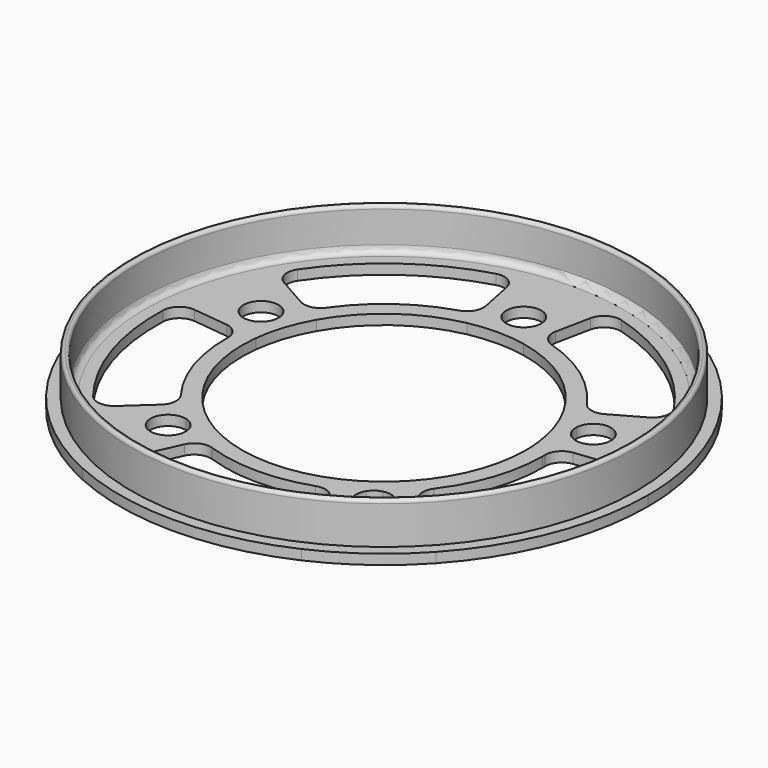
from build123d import *

# Parameters (mm, degrees)
F1_DEPTH = 3
F2_R     = 5
F3_R     = 75.6
F3_R_2   = 73.6
F4_DEPTH = 12.4
F5_R     = 0.99999
F6_R     = 2


# Not quite as in the source:
# - a fillet or chamfer is up to 0.001 mm smaller than in the source, because OpenCascade refuses the exact size


with BuildPart() as f1:
    # F0 (on Top) → F1 (new body)
    with BuildSketch(Plane.XY):
        with BuildLine():
            ThreePointArc((-13.5579196876, 66.6346967709), (0, 68), (13.5579196876, 66.6346967709))
            Line((13.5579196876, 66.6346967709), (15.7511125782, 77.4138388956))
            ThreePointArc((15.7511125782, 77.4138388956), (0, 79), (-15.7511125782, 77.4138388956))
            Line((-15.7511125782, 77.4138388956), (-13.5579196876, 66.6346967709))
        make_face()
        with BuildLine():
            ThreePointArc((13.5579196876, 66.6346967709), (39.9693971559, 55.0131556175), (59.1837349834, 33.4856015835))
            Line((59.1837349834, 33.4856015835), (68.7575744661, 38.902390075))
            ThreePointArc((68.7575744661, 38.902390075), (46.4350349311, 63.9123425556), (15.7511125782, 77.4138388956))
            Line((15.7511125782, 77.4138388956), (13.5579196876, 66.6346967709))
        make_face()
        with BuildLine():
            ThreePointArc((8.4736998047, 41.6466854818), (24.9808732224, 34.3832222609), (36.9898343647, 20.9285009897))
            Line((36.9898343647, 20.9285009897), (41.341579584, 23.3906775767))
            ThreePointArc((41.341579584, 23.3906775767), (27.9197994839, 38.4283072328), (9.4706056641, 46.5462955385))
            Line((9.4706056641, 46.5462955385), (8.4736998047, 41.6466854818))
        make_face()
        with BuildLine():
            ThreePointArc((-8.4736998047, 41.6466854818), (0, 42.5), (8.4736998047, 41.6466854818))
            Line((8.4736998047, 41.6466854818), (9.4706056641, 46.5462955385))
            ThreePointArc((9.4706056641, 46.5462955385), (5.7500684223, 47.1506809404), (1.9933228139, 47.4581569823))
            ThreePointArc((1.9933228139, 47.4581569823), (0, 47.0650247137), (-1.9933228139, 47.4581569823))
            ThreePointArc((-1.9933228139, 47.4581569823), (-5.7500684223, 47.1506809404), (-9.4706056641, 46.5462955385))
            Line((-9.4706056641, 46.5462955385), (-8.4736998047, 41.6466854818))
        make_face()
        with BuildLine():
            ThreePointArc((1.9933228139, 47.4581569823), (5.7500684223, 47.1506809404), (9.4706056641, 46.5462955385))
            Line((9.4706056641, 46.5462955385), (13.5579196876, 66.6346967709))
            ThreePointArc((13.5579196876, 66.6346967709), (0, 68), (-13.5579196876, 66.6346967709))
            Line((-13.5579196876, 66.6346967709), (-9.4706056641, 46.5462955385))
            ThreePointArc((-9.4706056641, 46.5462955385), (-5.7500684223, 47.1506809404), (-1.9933228139, 47.4581569823))
            ThreePointArc((-1.9933228139, 47.4581569823), (-2.9238292723, 56.6754974388), (5.25, 52.3150247137))
            ThreePointArc((5.25, 52.3150247137), (4.3604727251, 49.3911954414), (1.9933228139, 47.4581569823))
        make_face()
        with BuildLine():
            ThreePointArc((45.7513600742, 12.769614378), (46.6198312174, 9.1017216648), (47.1947357785, 5.3765151165))
            Line((47.1947357785, 5.3765151165), (67.5629901671, 7.6969058509))
            ThreePointArc((67.5629901671, 7.6969058509), (64.6718431081, 21.0131556175), (59.1837349834, 33.4856015835))
            Line((59.1837349834, 33.4856015835), (41.341579584, 23.3906775767))
            ThreePointArc((41.341579584, 23.3906775767), (43.0660934948, 20.039001749), (44.5194188246, 16.5611396805))
            ThreePointArc((44.5194188246, 16.5611396805), (49.952139145, 21.4125119623), (55.0045451541, 16.1662316977))
            ThreePointArc((55.0045451541, 16.1662316977), (51.5636579657, 11.2377825669), (45.7513600742, 12.769614378))
        make_face()
        with BuildLine():
            ThreePointArc((36.9898343647, 20.9285009897), (40.4199019425, 13.1332222609), (42.2268688544, 4.8105661568))
            Line((42.2268688544, 4.8105661568), (47.1947357785, 5.3765151165))
            ThreePointArc((47.1947357785, 5.3765151165), (46.6198312174, 9.1017216648), (45.7513600742, 12.769614378))
            ThreePointArc((45.7513600742, 12.769614378), (44.7614984435, 14.5438924772), (44.5194188246, 16.5611396805))
            ThreePointArc((44.5194188246, 16.5611396805), (43.0660934948, 20.039001749), (41.341579584, 23.3906775767))
            Line((41.341579584, 23.3906775767), (36.9898343647, 20.9285009897))
        make_face()
        with BuildLine():
            ThreePointArc((59.1837349834, 33.4856015835), (64.6718431081, 21.0131556175), (67.5629901671, 7.6969058509))
            Line((67.5629901671, 7.6969058509), (78.4922974, 8.9419935621))
            ThreePointArc((78.4922974, 8.9419935621), (75.1334647873, 24.4123425556), (68.7575744661, 38.902390075))
            Line((68.7575744661, 38.902390075), (59.1837349834, 33.4856015835))
        make_face()
        with BuildLine():
            Line((78.4922974, 8.9419935621), (67.5629901671, 7.6969058509))
            ThreePointArc((67.5629901671, 7.6969058509), (67.890659635, 3.8546509982), (68, 0))
            ThreePointArc((68, 0), (63.3767015757, -24.6453585365), (50.1354794885, -45.9394568585))
            Line((50.1354794885, -45.9394568585), (58.2456305823, -53.3708395856))
            ThreePointArc((58.2456305823, -53.3708395856), (73.6288150658, -28.6321077115), (79, 0))
            ThreePointArc((79, 0), (78.8729722231, 4.4781974832), (78.4922974, 8.9419935621))
        make_face()
        with BuildLine():
            ThreePointArc((42.2268688544, 4.8105661568), (42.4316622719, 2.4091568739), (42.5, 0))
            ThreePointArc((42.5, 0), (39.6104384848, -15.4033490853), (31.3346746803, -28.7121605366))
            Line((31.3346746803, -28.7121605366), (35.0211069957, -32.0900617762))
            ThreePointArc((35.0211069957, -32.0900617762), (44.2704900712, -17.2155078012), (47.5, 0))
            ThreePointArc((47.5, 0), (47.4236225392, 2.6925870943), (47.1947357785, 5.3765151165))
            Line((47.1947357785, 5.3765151165), (42.2268688544, 4.8105661568))
        make_face()
        with BuildLine():
            Line((35.0211069957, -32.0900617762), (31.3346746803, -28.7121605366))
            ThreePointArc((31.3346746803, -28.7121605366), (24.9808732224, -34.3832222609), (17.6239403858, -38.6735920917))
            Line((17.6239403858, -38.6735920917), (19.6973451371, -43.2234264555))
            ThreePointArc((19.6973451371, -43.2234264555), (23.0625718199, -41.5255075954), (26.2825727435, -39.5661012735))
            ThreePointArc((26.2825727435, -39.5661012735), (27.6641274255, -38.076404834), (29.5078368069, -37.2228097673))
            ThreePointArc((29.5078368069, -37.2228097673), (32.3663779647, -34.7658967588), (35.0211069957, -32.0900617762))
        make_face()
        with BuildLine():
            Line((19.6973451371, -43.2234264555), (17.6239403858, -38.6735920917))
            ThreePointArc((17.6239403858, -38.6735920917), (0, -42.5), (-17.6239403858, -38.6735920917))
            Line((-17.6239403858, -38.6735920917), (-19.6973451371, -43.2234264555))
            ThreePointArc((-19.6973451371, -43.2234264555), (0, -47.5), (19.6973451371, -43.2234264555))
        make_face()
        with BuildLine():
            ThreePointArc((-17.6239403858, -38.6735920917), (-24.9808732224, -34.3832222609), (-31.3346746803, -28.7121605366))
            Line((-31.3346746803, -28.7121605366), (-35.0211069957, -32.0900617762))
            ThreePointArc((-35.0211069957, -32.0900617762), (-32.3663779647, -34.7658967588), (-29.5078368069, -37.2228097673))
            ThreePointArc((-29.5078368069, -37.2228097673), (-27.6641274255, -38.076404834), (-26.2825727435, -39.5661012735))
            ThreePointArc((-26.2825727435, -39.5661012735), (-23.0625718199, -41.5255075954), (-19.6973451371, -43.2234264555))
            Line((-19.6973451371, -43.2234264555), (-17.6239403858, -38.6735920917))
        make_face()
        with BuildLine():
            Line((-35.0211069957, -32.0900617762), (-31.3346746803, -28.7121605366))
            ThreePointArc((-31.3346746803, -28.7121605366), (-40.4199019425, -13.1332222609), (-42.2268688544, 4.8105661568))
            Line((-42.2268688544, 4.8105661568), (-47.1947357785, 5.3765151165))
            ThreePointArc((-47.1947357785, 5.3765151165), (-45.175184524, -14.6783072328), (-35.0211069957, -32.0900617762))
        make_face()
        with BuildLine():
            ThreePointArc((-42.2268688544, 4.8105661568), (-40.4199019425, 13.1332222609), (-36.9898343647, 20.9285009897))
            Line((-36.9898343647, 20.9285009897), (-41.341579584, 23.3906775767))
            ThreePointArc((-41.341579584, 23.3906775767), (-43.0660934948, 20.039001749), (-44.5194188246, 16.5611396805))
            ThreePointArc((-44.5194188246, 16.5611396805), (-44.5082648895, 16.3638256886), (-44.5045451541, 16.1662316977))
            ThreePointArc((-44.5045451541, 16.1662316977), (-44.8260960233, 14.357118886), (-45.7513600742, 12.769614378))
            ThreePointArc((-45.7513600742, 12.769614378), (-46.6198312174, 9.1017216648), (-47.1947357785, 5.3765151165))
            Line((-47.1947357785, 5.3765151165), (-42.2268688544, 4.8105661568))
        make_face()
        with BuildLine():
            Line((-41.341579584, 23.3906775767), (-36.9898343647, 20.9285009897))
            ThreePointArc((-36.9898343647, 20.9285009897), (-24.9808732224, 34.3832222609), (-8.4736998047, 41.6466854818))
            Line((-8.4736998047, 41.6466854818), (-9.4706056641, 46.5462955385))
            ThreePointArc((-9.4706056641, 46.5462955385), (-27.9197994839, 38.4283072328), (-41.341579584, 23.3906775767))
        make_face()
        with BuildLine():
            ThreePointArc((-44.5194188246, 16.5611396805), (-43.0660934948, 20.039001749), (-41.341579584, 23.3906775767))
            Line((-41.341579584, 23.3906775767), (-59.1837349834, 33.4856015835))
            ThreePointArc((-59.1837349834, 33.4856015835), (-64.6718431081, 21.0131556175), (-67.5629901671, 7.6969058509))
            Line((-67.5629901671, 7.6969058509), (-47.1947357785, 5.3765151165))
            ThreePointArc((-47.1947357785, 5.3765151165), (-46.6198312174, 9.1017216648), (-45.7513600742, 12.769614378))
            ThreePointArc((-45.7513600742, 12.769614378), (-54.7475918646, 17.7885709181), (-44.5194188246, 16.5611396805))
        make_face()
        with BuildLine():
            ThreePointArc((-67.5629901671, 7.6969058509), (-64.6718431081, 21.0131556175), (-59.1837349834, 33.4856015835))
            Line((-59.1837349834, 33.4856015835), (-68.7575744661, 38.902390075))
            ThreePointArc((-68.7575744661, 38.902390075), (-75.1334647873, 24.4123425556), (-78.4922974, 8.9419935621))
            Line((-78.4922974, 8.9419935621), (-67.5629901671, 7.6969058509))
        make_face()
        with BuildLine():
            ThreePointArc((-28.1983046173, -61.8777473468), (-39.9693971559, -55.0131556175), (-50.1354794885, -45.9394568585))
            Line((-50.1354794885, -45.9394568585), (-58.2456305823, -53.3708395856))
            ThreePointArc((-58.2456305823, -53.3708395856), (-46.4350349311, -63.9123425556), (-32.7597950701, -71.887382947))
            Line((-32.7597950701, -71.887382947), (-28.1983046173, -61.8777473468))
        make_face()
        with BuildLine():
            ThreePointArc((-29.5078368069, -37.2228097673), (-32.3663779647, -34.7658967588), (-35.0211069957, -32.0900617762))
            Line((-35.0211069957, -32.0900617762), (-50.1354794885, -45.9394568585))
            ThreePointArc((-50.1354794885, -45.9394568585), (-39.9693971559, -55.0131556175), (-28.1983046173, -61.8777473468))
            Line((-28.1983046173, -61.8777473468), (-19.6973451371, -43.2234264555))
            ThreePointArc((-19.6973451371, -43.2234264555), (-23.0625718199, -41.5255075954), (-26.2825727435, -39.5661012735))
            ThreePointArc((-26.2825727435, -39.5661012735), (-25.6994310669, -40.8904773481), (-25.5, -42.3237440545))
            ThreePointArc((-25.5, -42.3237440545), (-34.8781870575, -45.5672871201), (-29.5078368069, -37.2228097673))
        make_face()
        with BuildLine():
            Line((-58.2456305823, -53.3708395856), (-50.1354794885, -45.9394568585))
            ThreePointArc((-50.1354794885, -45.9394568585), (-64.6718431081, -21.0131556175), (-67.5629901671, 7.6969058509))
            Line((-67.5629901671, 7.6969058509), (-78.4922974, 8.9419935621))
            ThreePointArc((-78.4922974, 8.9419935621), (-75.1334647873, -24.4123425556), (-58.2456305823, -53.3708395856))
        make_face()
        with BuildLine():
            Line((-68.7575744661, 38.902390075), (-59.1837349834, 33.4856015835))
            ThreePointArc((-59.1837349834, 33.4856015835), (-39.9693971559, 55.0131556175), (-13.5579196876, 66.6346967709))
            Line((-13.5579196876, 66.6346967709), (-15.7511125782, 77.4138388956))
            ThreePointArc((-15.7511125782, 77.4138388956), (-46.4350349311, 63.9123425556), (-68.7575744661, 38.902390075))
        make_face()
        with BuildLine():
            Line((32.7597950701, -71.887382947), (28.1983046173, -61.8777473468))
            ThreePointArc((28.1983046173, -61.8777473468), (0, -68), (-28.1983046173, -61.8777473468))
            Line((-28.1983046173, -61.8777473468), (-32.7597950701, -71.887382947))
            ThreePointArc((-32.7597950701, -71.887382947), (0, -79), (32.7597950701, -71.887382947))
        make_face()
        with BuildLine():
            Line((58.2456305823, -53.3708395856), (50.1354794885, -45.9394568585))
            ThreePointArc((50.1354794885, -45.9394568585), (39.9693971559, -55.0131556175), (28.1983046173, -61.8777473468))
            Line((28.1983046173, -61.8777473468), (32.7597950701, -71.887382947))
            ThreePointArc((32.7597950701, -71.887382947), (46.4350349311, -63.9123425556), (58.2456305823, -53.3708395856))
        make_face()
        with BuildLine():
            Line((50.1354794885, -45.9394568585), (35.0211069957, -32.0900617762))
            ThreePointArc((35.0211069957, -32.0900617762), (32.3663779647, -34.7658967588), (29.5078368069, -37.2228097673))
            ThreePointArc((29.5078368069, -37.2228097673), (33.9935430656, -38.195556997), (36, -42.3237440545))
            ThreePointArc((36, -42.3237440545), (29.3167332936, -47.3743129876), (26.2825727435, -39.5661012735))
            ThreePointArc((26.2825727435, -39.5661012735), (23.0625718199, -41.5255075954), (19.6973451371, -43.2234264555))
            Line((19.6973451371, -43.2234264555), (28.1983046173, -61.8777473468))
            ThreePointArc((28.1983046173, -61.8777473468), (39.9693971559, -55.0131556175), (50.1354794885, -45.9394568585))
        make_face()
    extrude(amount=F1_DEPTH)

    # F2
    f2_edges = [f1.edges().sort_by_distance(p)[0] for p in [
        (13.55792, 66.634697, 1.5),
        (59.183735, 33.485602, 1.5),
        (41.34158, 23.390678, 1.5),
        (9.470606, 46.546296, 1.5),
        (35.021107, -32.090062, 1.5),
        (47.194736, 5.376515, 1.5),
        (67.56299, 7.696906, 1.5),
        (-13.55792, 66.634697, 1.5),
        (50.135479, -45.939457, 1.5),
        (28.198305, -61.877747, 1.5),
        (19.697345, -43.223426, 1.5),
        (-47.194736, 5.376515, 1.5),
        (-35.021107, -32.090062, 1.5),
        (-19.697345, -43.223426, 1.5),
        (-28.198305, -61.877747, 1.5),
        (-50.135479, -45.939457, 1.5),
        (-67.56299, 7.696906, 1.5),
        (-59.183735, 33.485602, 1.5),
        (-41.34158, 23.390678, 1.5),
        (-9.470606, 46.546296, 1.5),
    ]]
    fillet(f2_edges, radius=F2_R)

    # F3 (on face) → F4 (join)
    with BuildSketch(Plane.XY.offset(3)):
        Circle(F3_R)
        Circle(F3_R_2, mode=Mode.SUBTRACT)
    extrude(amount=F4_DEPTH)

    # F5 (radius 1 in the source; OpenCascade refuses exactly that, so slightly less here)
    f5_edges = [f1.edges().sort_by_distance(p)[0] for p in [
        (-75.6, 0, 15.4),
        (-73.6, 0, 15.4),
    ]]
    fillet(f5_edges, radius=F5_R)

    # F6
    f6_edges = [f1.edges().sort_by_distance(p)[0] for p in [
        (-73.6, 0, 3),
    ]]
    fillet(f6_edges, radius=F6_R)


solid = f1.part
